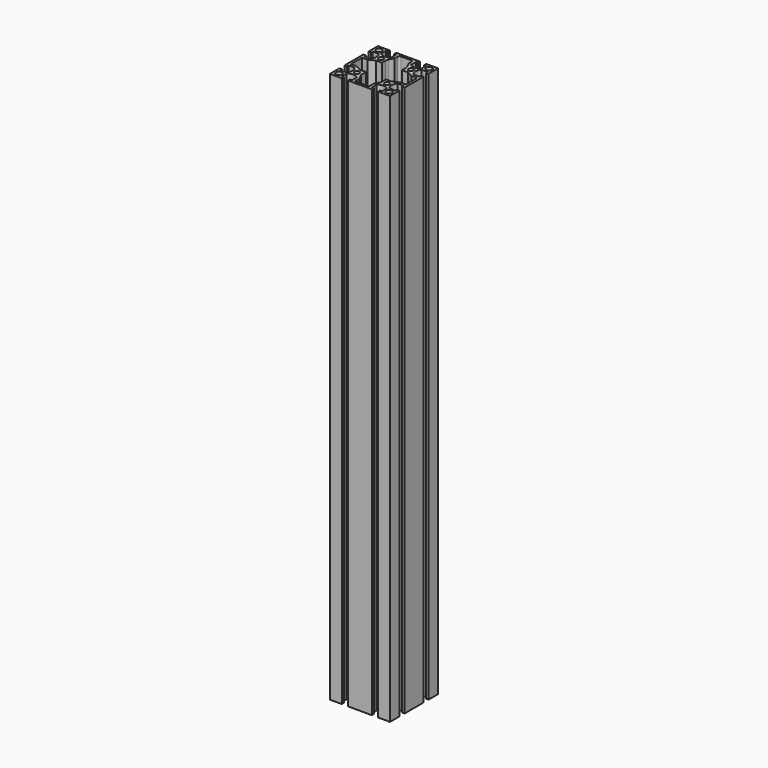
from build123d import *

# Parameters (mm, degrees)
F0_R     = 3
F0_R_2   = 2.5
F1_DEPTH = 550
F2_R     = 2
F3_R     = 7


# Not quite as in the source:
# - a feature names something its author has since deleted; it is built from what else it names


with BuildPart() as f1:
    # F0 (on Top) → F1 (new body)
    with BuildSketch(Plane.XY):
        with BuildLine():
            Line((18.15, -30), (30, -30))
            Line((30, -30), (30, -18.15))
            Line((30, -18.15), (27.5, -18.15))
            Line((27.5, -18.15), (27.5, -20.15))
            Line((27.5, -20.15), (21.5477069044, -20.15))
            ThreePointArc((21.5477069044, -20.15), (19.5, -15), (21.5477069044, -9.85))
            Line((21.5477069044, -9.85), (27.5, -9.85))
            Line((27.5, -9.85), (27.5, -11.85))
            Line((27.5, -11.85), (30, -11.85))
            Line((30, -11.85), (30, 11.85))
            Line((30, 11.85), (27.5, 11.85))
            Line((27.5, 11.85), (27.5, 9.85))
            Line((27.5, 9.85), (21.5477069044, 9.85))
            ThreePointArc((21.5477069044, 9.85), (19.5, 15), (21.5477069044, 20.15))
            Line((21.5477069044, 20.15), (27.5, 20.15))
            Line((27.5, 20.15), (27.5, 18.15))
            Line((27.5, 18.15), (30, 18.15))
            Line((30, 18.15), (30, 30))
            Line((30, 30), (18.15, 30))
            Line((18.15, 30), (18.15, 27.5))
            Line((18.15, 27.5), (20.15, 27.5))
            Line((20.15, 27.5), (20.15, 21.5477069044))
            ThreePointArc((20.15, 21.5477069044), (15, 19.5), (9.85, 21.5477069044))
            Line((9.85, 21.5477069044), (9.85, 27.5))
            Line((9.85, 27.5), (11.85, 27.5))
            Line((11.85, 27.5), (11.85, 30))
            Line((11.85, 30), (-11.85, 30))
            Line((-11.85, 30), (-11.85, 27.5))
            Line((-11.85, 27.5), (-9.85, 27.5))
            Line((-9.85, 27.5), (-9.85, 21.5477069044))
            ThreePointArc((-9.85, 21.5477069044), (-15, 19.5), (-20.15, 21.5477069044))
            Line((-20.15, 21.5477069044), (-20.15, 27.5))
            Line((-20.15, 27.5), (-18.15, 27.5))
            Line((-18.15, 27.5), (-18.15, 30))
            Line((-18.15, 30), (-30, 30))
            Line((-30, 30), (-30, 18.15))
            Line((-30, 18.15), (-27.5, 18.15))
            Line((-27.5, 18.15), (-27.5, 20.15))
            Line((-27.5, 20.15), (-21.5477069044, 20.15))
            ThreePointArc((-21.5477069044, 20.15), (-19.5, 15), (-21.5477069044, 9.85))
            Line((-21.5477069044, 9.85), (-27.5, 9.85))
            Line((-27.5, 9.85), (-27.5, 11.85))
            Line((-27.5, 11.85), (-30, 11.85))
            Line((-30, 11.85), (-30, -11.85))
            Line((-30, -11.85), (-27.5, -11.85))
            Line((-27.5, -11.85), (-27.5, -9.85))
            Line((-27.5, -9.85), (-21.5477069044, -9.85))
            ThreePointArc((-21.5477069044, -9.85), (-19.5, -15), (-21.5477069044, -20.15))
            Line((-21.5477069044, -20.15), (-27.5, -20.15))
            Line((-27.5, -20.15), (-27.5, -18.15))
            Line((-27.5, -18.15), (-30, -18.15))
            Line((-30, -18.15), (-30, -30))
            Line((-30, -30), (-18.15, -30))
            Line((-18.15, -30), (-18.15, -27.5))
            Line((-18.15, -27.5), (-20.15, -27.5))
            Line((-20.15, -27.5), (-20.15, -21.5477069044))
            ThreePointArc((-20.15, -21.5477069044), (-15, -19.5), (-9.85, -21.5477069044))
            Line((-9.85, -21.5477069044), (-9.85, -27.5))
            Line((-9.85, -27.5), (-11.85, -27.5))
            Line((-11.85, -27.5), (-11.85, -30))
            Line((-11.85, -30), (11.85, -30))
            Line((11.85, -30), (11.85, -27.5))
            Line((11.85, -27.5), (9.85, -27.5))
            Line((9.85, -27.5), (9.85, -21.5477069044))
            ThreePointArc((9.85, -21.5477069044), (15, -19.5), (20.15, -21.5477069044))
            Line((20.15, -21.5477069044), (20.15, -27.5))
            Line((20.15, -27.5), (18.15, -27.5))
            Line((18.15, -27.5), (18.15, -30))
        make_face()
        with Locations((-25, -25)):
            Circle(F0_R, mode=Mode.SUBTRACT)
        with Locations((-15, -15)):
            Circle(F0_R_2, mode=Mode.SUBTRACT)
        with Locations((25, -25)):
            Circle(F0_R, mode=Mode.SUBTRACT)
        with Locations((15, -15)):
            Circle(F0_R_2, mode=Mode.SUBTRACT)
        with Locations((-25, 25)):
            Circle(F0_R, mode=Mode.SUBTRACT)
        with Locations((-15, 15)):
            Circle(F0_R_2, mode=Mode.SUBTRACT)
        Polygon((-7, 22), (-7, 27.5), (0, 27.5), (7, 27.5), (7, 22), (10, 16), (10, 10), (16, 10), (22, 7), (27.5, 7), (27.5, 0), (27.5, -7), (22, -7), (16, -10), (10, -10), (10, -16), (7, -22), (7, -27.5), (0, -27.5), (-7, -27.5), (-7, -22), (-10, -16), (-10, -10), (-16, -10), (-22, -7), (-27.5, -7), (-27.5, 0), (-27.5, 7), (-22, 7), (-16, 10), (-10, 10), (-10, 16), align=None, mode=Mode.SUBTRACT)
        with Locations((15, 15)):
            Circle(F0_R_2, mode=Mode.SUBTRACT)
        with Locations((25, 25)):
            Circle(F0_R, mode=Mode.SUBTRACT)
    extrude(amount=F1_DEPTH)

    # F2
    f2_edges = [f1.edges().sort_by_distance(p)[0] for p in [
        (-7, 27.5, 275),
        (7, 27.5, 275),
    ]]
    fillet(f2_edges, radius=F2_R)

    # F3
    f3_edges = [f1.edges().sort_by_distance(p)[0] for p in [
        (-10, 16, 275),
        (10, 16, 275),
    ]]
    fillet(f3_edges, radius=F3_R)


solid = f1.part
